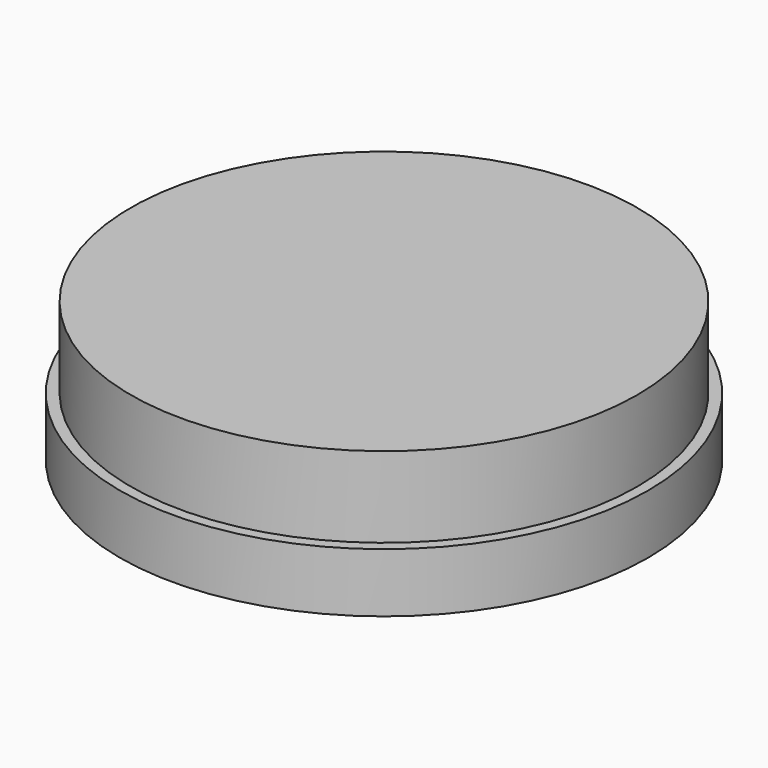
from build123d import *

# Parameters (mm, degrees)
F0_W   = 0.2
F0_H   = 1.1
F0_W_2 = 0.8
F0_H_2 = 1.5


# Not quite as in the source:
# - a feature names something its author has since deleted; it is built from what else it names


with BuildPart() as f1:
    # F0 (on Front) → F1 (revolve)
    with BuildSketch(Plane.XZ):
        Polygon((4.71, 2.6), (0, 2.6), (0, 1.5), (1.21, 1.5), (2.01, 1.5), (3.91, 1.5), (3.91, 1.1), (3.91, 0), (4.71, 0), (4.71, 1.1), align=None)
        with Locations((4.81, 0.55)):
            Rectangle(F0_W, F0_H)
        with Locations((3.81, 0.55)):
            Rectangle(F0_W, F0_H)
        with Locations((1.61, 0.75)):
            Rectangle(F0_W_2, F0_H_2)
    revolve(axis=Axis((0, 0, 1.3), (0, 0, 1)))


solid = f1.part
